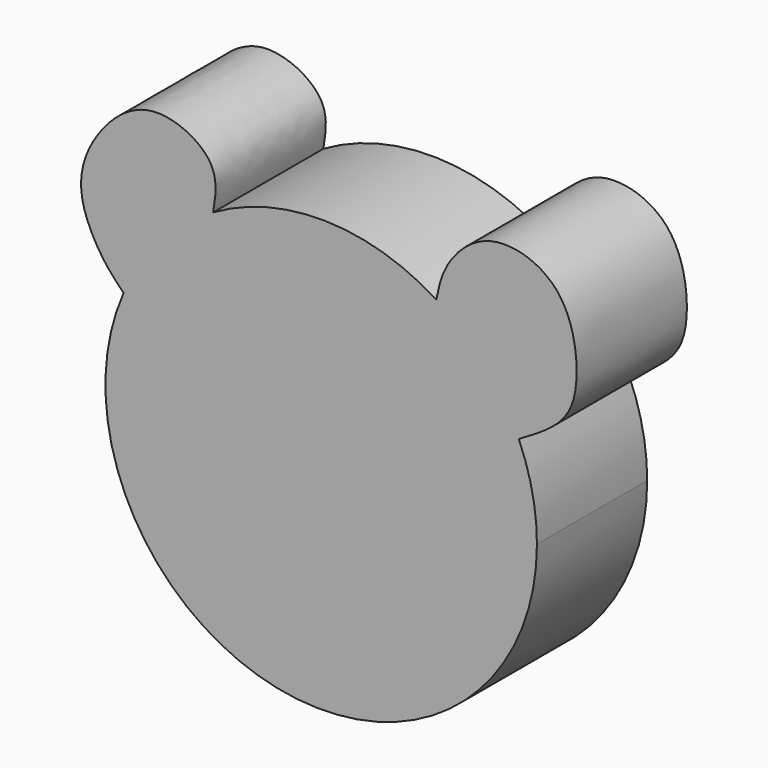
from build123d import *

# Parameters (mm, degrees)
F2_DEPTH = 17.78


# Not quite as in the source:
# - the program builds the solid bodies; features that only make, move or delete a surface that nothing else refers to are left out


with BuildPart() as f2:
    # F0 (on Front) → F2 (new body)
    with BuildSketch(Plane.XZ):
        with BuildLine():
            ThreePointArc((-25.4854624617, 11.1814313142), (-5.7123399341, -27.2378849325), (27.8304366318, 0))
            ThreePointArc((27.8304366318, 0), (27.2378849325, 5.7123399341), (25.4854624617, 11.1814313142))
            ThreePointArc((25.4854624617, 11.1814313142), (21.0894268244, 18.1595506369), (14.8413239123, 23.5429035518))
            ThreePointArc((14.8413239123, 23.5429035518), (0.5278354358, 27.8254306862), (-13.9377721615, 24.088829575))
            ThreePointArc((-13.9377721615, 24.088829575), (-20.7412171654, 18.5562688495), (-25.4854624617, 11.1814313142))
        make_face()
        with BuildLine():
            ThreePointArc((14.8413239123, 23.5429035518), (21.0894268244, 18.1595506369), (25.4854624617, 11.1814313142))
            add(Edge.make_bspline(
                [(14.8413239123, 23.5429035518), (15.1413649797, 25.0040188999), (15.7986912782, 28.260631254), (21.5932657669, 34.1059217282), (32.0206442284, 30.9740164086), (33.5512212932, 20.0305004366), (31.4640007875, 14.6491656343), (27.5467324966, 12.3770350557), (25.4854624617, 11.1814313142)],
                knots=[0, 0, 0, 0, 0.1361039331, 0.3050174671, 0.492706302, 0.690645138, 0.8373233948, 1, 1, 1, 1], degree=3))
        make_face()
        with BuildLine():
            add(Edge.make_bspline(
                [(-13.9377721615, 24.088829575), (-13.6149779351, 26.0443059259), (-12.9059851741, 30.3443635616), (-22.1612583852, 34.9079889108), (-29.3313166227, 28.6211389756), (-32.0623724786, 21.0496503131), (-28.3666845132, 14.0775517686), (-26.3518766449, 12.0465521212), (-25.4854624617, 11.1814313142)],
                knots=[0, 0, 0, 0, 0.1517157978, 0.3337238633, 0.5207376803, 0.6981342072, 0.871564045, 1, 1, 1, 1], degree=3))
            ThreePointArc((-25.4854624617, 11.1814313142), (-20.7412171654, 18.5562688495), (-13.9377721615, 24.088829575))
        make_face()
    extrude(amount=F2_DEPTH)


solid = f2.part
